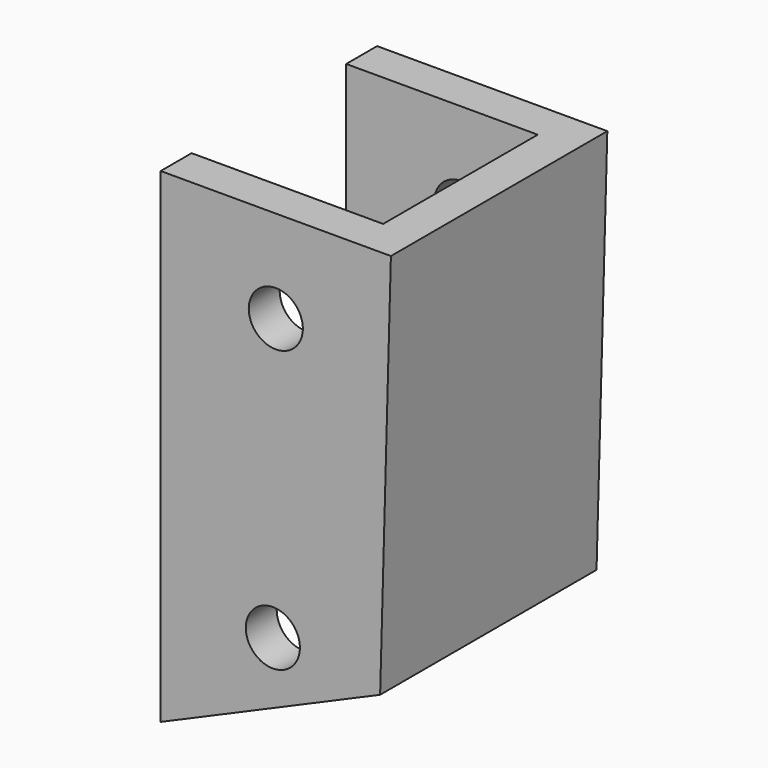
from build123d import *

# Parameters (mm, degrees)
F1_DEPTH = 8.89
F2_T     = -1.27
F3_D     = 1.778


# Not quite as in the source:
# - a feature names something its author has since deleted; it is built from what else it names


with BuildPart() as f1:
    # F0 (on Front) → F1 (new body)
    with BuildSketch(Plane.XZ):
        Polygon((-45.8687357605, 33.5707478225), (-45.5147512257, 46.3788583875), (-53.0798770487, 46.3788583875), (-53.0798770487, 30.4408613592), align=None)
    extrude(amount=F1_DEPTH)

    # F2
    f2_openings = [f1.faces().sort_by_distance(p)[0] for p in [
        (-49.297314, -4.445, 46.378858),
        (-53.079877, -4.445, 38.40986),
        (-49.474306, -4.445, 32.005805),
    ]]
    offset(amount=F2_T, openings=f2_openings)

    # F3 (through all)
    with Locations(Plane(origin=(0, 0, 0), x_dir=(1, 0, 0), z_dir=(0, 1, 0))):
        with Locations((-49.2973141372, -43.3367788792), (-49.3943579495, -34.0744107962)):
            Hole(F3_D / 2)


solid = f1.part
